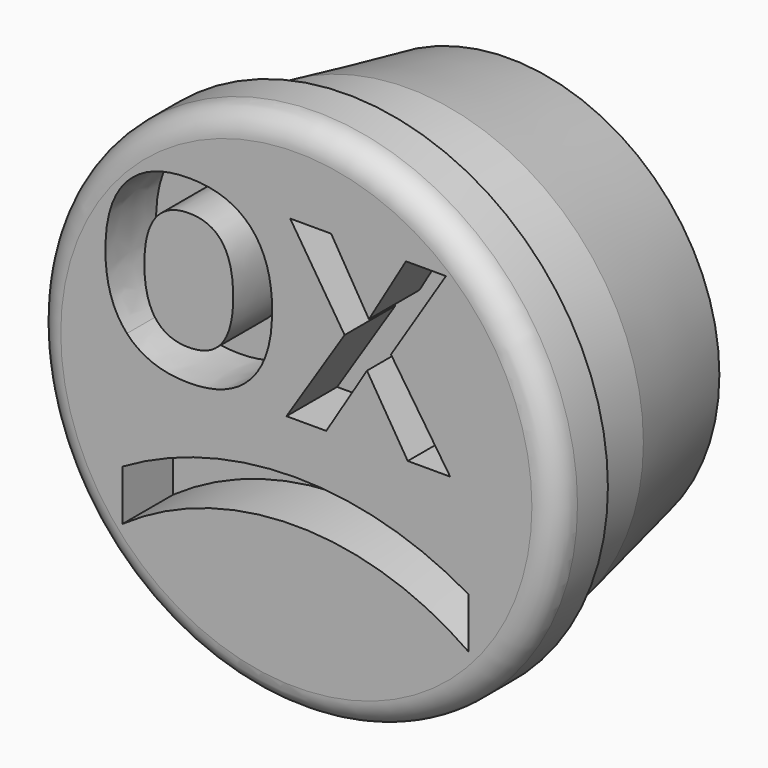
from build123d import *

# Parameters (mm, degrees)
F1_DEPTH     = 3.175
F0_R         = 13.081
F0_R_2       = 11.811
F0_TEXT_SIZE = 12.3047218141
F2_DEPTH     = 10.16
F3_R         = 1.27
F4_SIZE2     = 1.27
F4_SIZE      = 6.35


# Not quite as in the source:
# - Text() gives the source's letters only with a copy of the font that has no kerning and outlines rounded to 1/6400 em; it was checked with that copy


with BuildPart() as f1:
    # F0 (on Front) → F1 (new body)
    with BuildSketch(Plane.XZ):
        with BuildLine():
            add(Edge.make_bspline(
                [(-7.0565526427, 6.623401039), (-7.6208394946, 5.8755046662), (-7.6208394946, 4.4047058869)],
                knots=[0, 0, 0, 1, 1, 1], degree=2))
            add(Edge.make_bspline(
                [(-7.6208394946, 4.4047058869), (-7.6208394946, 2.9319844948), (-7.0623204811, 2.1869720412)],
                knots=[0, 0, 0, 1, 1, 1], degree=2))
            add(Edge.make_bspline(
                [(-7.0623204811, 2.1869720412), (-6.5038014675, 1.4419595876), (-5.3925312786, 1.4419595876)],
                knots=[0, 0, 0, 1, 1, 1], degree=2))
            add(Edge.make_bspline(
                [(-5.3925312786, 1.4419595876), (-3.1642230626, 1.4419595876), (-3.1642230626, 4.4047058869)],
                knots=[0, 0, 0, 1, 1, 1], degree=2))
            add(Edge.make_bspline(
                [(-3.1642230626, 4.4047058869), (-3.1642230626, 7.3712974117), (-5.3809956019, 7.3712974117)],
                knots=[0, 0, 0, 1, 1, 1], degree=2))
            add(Edge.make_bspline(
                [(-5.3809956019, 7.3712974117), (-6.4922657908, 7.3712974117), (-7.0565526427, 6.623401039)],
                knots=[0, 0, 0, 1, 1, 1], degree=2))
        make_face()
    extrude(amount=F1_DEPTH)


with BuildPart() as f1b:
    # F0 (on Front) → F1, piece 2 (new body)
    with BuildSketch(Plane.XZ):
        Circle(F0_R)
        Circle(F0_R_2, mode=Mode.SUBTRACT)
        Circle(F0_R_2)
        with BuildLine():
            ThreePointArc((-8.715332835, -4.8949569879), (-0.039609964, -2.5486091617), (8.636112907, -4.8949569879))
            Line((8.636112907, -4.8949569879), (8.636112907, -7.4279978871))
            ThreePointArc((8.636112907, -7.4279978871), (-0.039609964, -4.6822091414), (-8.715332835, -7.4279978871))
            Line((-8.715332835, -7.4279978871), (-8.715332835, -4.8949569879))
        make_face(mode=Mode.SUBTRACT)
        with BuildLine():
            add(Edge.make_bspline(
                [(-2.2836664078, 7.7567812748), (-1.2108484746, 6.5907166217), (-1.2108484746, 4.4047058869)],
                knots=[0, 0, 0, 1, 1, 1], degree=2))
            add(Edge.make_bspline(
                [(-1.2108484746, 4.4047058869), (-1.2108484746, 2.2225403777), (-2.2923181653, 1.0507078862)],
                knots=[0, 0, 0, 1, 1, 1], degree=2))
            add(Edge.make_bspline(
                [(-2.2923181653, 1.0507078862), (-3.373787856, -0.1211246054), (-5.3925312786, -0.1211246054)],
                knots=[0, 0, 0, 1, 1, 1], degree=2))
            add(Edge.make_bspline(
                [(-5.3925312786, -0.1211246054), (-7.4112747012, -0.1211246054), (-8.4927443919, 1.0507078862)],
                knots=[0, 0, 0, 1, 1, 1], degree=2))
            add(Edge.make_bspline(
                [(-8.4927443919, 1.0507078862), (-9.5742140826, 2.2225403777), (-9.5742140826, 4.4162415636)],
                knots=[0, 0, 0, 1, 1, 1], degree=2))
            add(Edge.make_bspline(
                [(-9.5742140826, 4.4162415636), (-9.5742140826, 6.6099427495), (-8.4898604728, 7.7663943387)],
                knots=[0, 0, 0, 1, 1, 1], degree=2))
            add(Edge.make_bspline(
                [(-8.4898604728, 7.7663943387), (-7.4055068629, 8.922845928), (-5.3809956019, 8.922845928)],
                knots=[0, 0, 0, 1, 1, 1], degree=2))
            add(Edge.make_bspline(
                [(-5.3809956019, 8.922845928), (-3.356484341, 8.922845928), (-2.2836664078, 7.7567812748)],
                knots=[0, 0, 0, 1, 1, 1], degree=2))
        make_face(mode=Mode.SUBTRACT)
        Polygon((4.7434833157, 4.4277772403), (7.7119974533, 0), (5.5855877149, 0), (3.541850326, 3.3222748898), (1.50003555, 0), (-0.4956365192, 0), (2.4190444605, 4.5296757178), (-0.3091430792, 8.7844178076), (1.7461299863, 8.7844178076), (3.6379809652, 5.6236423916), (5.495224914, 8.7844178076), (7.5005100472, 8.7844178076), align=None, mode=Mode.SUBTRACT)
    extrude(amount=F1_DEPTH)

    # F3
    f3_edges = [f1b.edges().sort_by_distance(p)[0] for p in [
        (-13.081, -3.175, 0),
    ]]
    fillet(f3_edges, radius=F3_R)


with BuildPart() as f2:
    # F0 (on Front) → F2 (new body)
    with BuildSketch(Plane.XZ):
        Circle(F0_R_2)
        with BuildLine():
            ThreePointArc((-8.715332835, -4.8949569879), (-0.039609964, -2.5486091617), (8.636112907, -4.8949569879))
            Line((8.636112907, -4.8949569879), (8.636112907, -7.4279978871))
            ThreePointArc((8.636112907, -7.4279978871), (-0.039609964, -4.6822091414), (-8.715332835, -7.4279978871))
            Line((-8.715332835, -7.4279978871), (-8.715332835, -4.8949569879))
        make_face(mode=Mode.SUBTRACT)
        with BuildLine():
            add(Edge.make_bspline(
                [(-2.2836664078, 7.7567812748), (-1.2108484746, 6.5907166217), (-1.2108484746, 4.4047058869)],
                knots=[0, 0, 0, 1, 1, 1], degree=2))
            add(Edge.make_bspline(
                [(-1.2108484746, 4.4047058869), (-1.2108484746, 2.2225403777), (-2.2923181653, 1.0507078862)],
                knots=[0, 0, 0, 1, 1, 1], degree=2))
            add(Edge.make_bspline(
                [(-2.2923181653, 1.0507078862), (-3.373787856, -0.1211246054), (-5.3925312786, -0.1211246054)],
                knots=[0, 0, 0, 1, 1, 1], degree=2))
            add(Edge.make_bspline(
                [(-5.3925312786, -0.1211246054), (-7.4112747012, -0.1211246054), (-8.4927443919, 1.0507078862)],
                knots=[0, 0, 0, 1, 1, 1], degree=2))
            add(Edge.make_bspline(
                [(-8.4927443919, 1.0507078862), (-9.5742140826, 2.2225403777), (-9.5742140826, 4.4162415636)],
                knots=[0, 0, 0, 1, 1, 1], degree=2))
            add(Edge.make_bspline(
                [(-9.5742140826, 4.4162415636), (-9.5742140826, 6.6099427495), (-8.4898604728, 7.7663943387)],
                knots=[0, 0, 0, 1, 1, 1], degree=2))
            add(Edge.make_bspline(
                [(-8.4898604728, 7.7663943387), (-7.4055068629, 8.922845928), (-5.3809956019, 8.922845928)],
                knots=[0, 0, 0, 1, 1, 1], degree=2))
            add(Edge.make_bspline(
                [(-5.3809956019, 8.922845928), (-3.356484341, 8.922845928), (-2.2836664078, 7.7567812748)],
                knots=[0, 0, 0, 1, 1, 1], degree=2))
        make_face(mode=Mode.SUBTRACT)
        Polygon((4.7434833157, 4.4277772403), (7.7119974533, 0), (5.5855877149, 0), (3.541850326, 3.3222748898), (1.50003555, 0), (-0.4956365192, 0), (2.4190444605, 4.5296757178), (-0.3091430792, 8.7844178076), (1.7461299863, 8.7844178076), (3.6379809652, 5.6236423916), (5.495224914, 8.7844178076), (7.5005100472, 8.7844178076), align=None, mode=Mode.SUBTRACT)
        with BuildLine():
            Line((8.636112907, -7.4279978871), (8.636112907, -4.8949569879))
            ThreePointArc((8.636112907, -4.8949569879), (-0.039609964, -2.5486091617), (-8.715332835, -4.8949569879))
            Line((-8.715332835, -4.8949569879), (-8.715332835, -7.4279978871))
            ThreePointArc((-8.715332835, -7.4279978871), (-0.039609964, -4.6822091414), (8.636112907, -7.4279978871))
        make_face()
        with Locations((-10.2894260381, 0)):
            Text('OX', F0_TEXT_SIZE, font='Open Sans', font_style=FontStyle.BOLD, text_align=(TextAlign.LEFT, TextAlign.BOTTOM))
        with BuildLine():
            add(Edge.make_bspline(
                [(-7.0565526427, 6.623401039), (-7.6208394946, 5.8755046662), (-7.6208394946, 4.4047058869)],
                knots=[0, 0, 0, 1, 1, 1], degree=2))
            add(Edge.make_bspline(
                [(-7.6208394946, 4.4047058869), (-7.6208394946, 2.9319844948), (-7.0623204811, 2.1869720412)],
                knots=[0, 0, 0, 1, 1, 1], degree=2))
            add(Edge.make_bspline(
                [(-7.0623204811, 2.1869720412), (-6.5038014675, 1.4419595876), (-5.3925312786, 1.4419595876)],
                knots=[0, 0, 0, 1, 1, 1], degree=2))
            add(Edge.make_bspline(
                [(-5.3925312786, 1.4419595876), (-3.1642230626, 1.4419595876), (-3.1642230626, 4.4047058869)],
                knots=[0, 0, 0, 1, 1, 1], degree=2))
            add(Edge.make_bspline(
                [(-3.1642230626, 4.4047058869), (-3.1642230626, 7.3712974117), (-5.3809956019, 7.3712974117)],
                knots=[0, 0, 0, 1, 1, 1], degree=2))
            add(Edge.make_bspline(
                [(-5.3809956019, 7.3712974117), (-6.4922657908, 7.3712974117), (-7.0565526427, 6.623401039)],
                knots=[0, 0, 0, 1, 1, 1], degree=2))
        make_face()
    extrude(amount=-F2_DEPTH)

    # F4
    f4_edges = [f2.edges().sort_by_distance(p)[0] for p in [
        (-11.811, 10.16, 0),
    ]]
    f4_side = f2.faces().sort_by_distance((-11.811, 5.08, 0))[0]
    chamfer(f4_edges, length=F4_SIZE, length2=F4_SIZE2, reference=f4_side)


solid = Compound([f1.part, f1b.part, f2.part])
